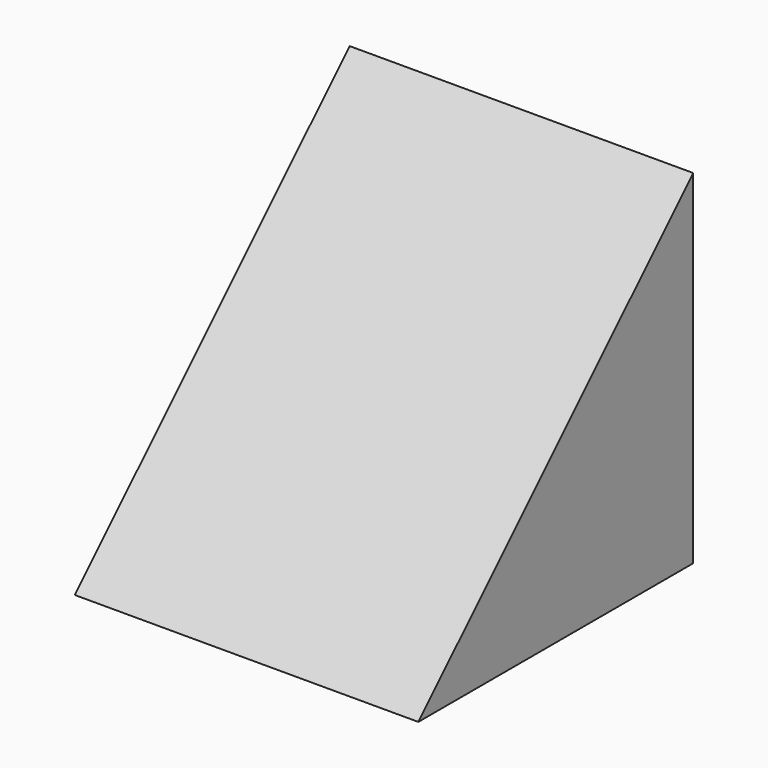
from build123d import *

# Parameters (mm, degrees)
F1_DEPTH = 3.175


# Not quite as in the source:
# - a feature names something its author has since deleted; it is built from what else it names


with BuildPart() as f1:
    # F0 (on Right) → F1 (new body, symmetric)
    with BuildSketch(Plane.YZ):
        Polygon((3.175, 3.175), (-3.175, -3.175), (3.175, -3.175), align=None)
    extrude(amount=F1_DEPTH, both=True)


solid = f1.part
